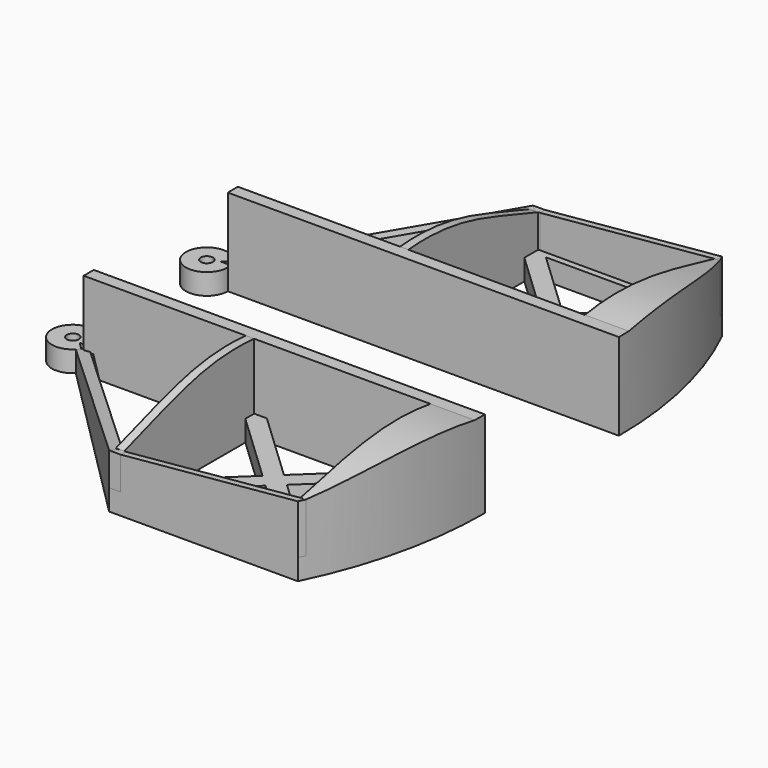
from build123d import *

# Parameters (mm, degrees)
F1_DEPTH       = 6.35
F2_R           = 1.8415
F3_DEPTH       = 25.4
F4_W           = 2.9205800795
F4_H           = 3.84
F5_DEPTH       = 20
F7_DEPTH       = 3.175
F9_DEPTH       = 1.905
F7_FACE_W      = 3.175
F7_FACE_H      = 10
F9_FACE_W      = 1.905
F9_FACE_H      = 10
F12_DEPTH      = 2.54
F16_END_RADIUS = 125
F15_W          = 3.84
F15_H          = 20
F16_REACH      = 136.0957238483
F18_DEPTH      = 15
F21_END_RADIUS = 125
F21_REACH      = 66.9646272281
F23_END_RADIUS = 125
F22_W          = 3.84
F22_H          = 20
F23_REACH      = 136.0957238483


with BuildPart() as f1:
    # F0 (on Top) → F1 (new body)
    with BuildSketch(Plane.XY):
        with BuildLine():
            Line((6.35, 0), (0, 0))
            Line((0, 0), (4.4901280605, 4.4901280605))
            ThreePointArc((4.4901280605, 4.4901280605), (-5.8666350314, -2.4300397955), (6.35, 0))
        make_face()
        with BuildLine():
            Line((4.4901280605, 4.4901280605), (0, 0))
            Line((0, 0), (6.35, 0))
            ThreePointArc((6.35, 0), (6.3162867067, 0.6534693866), (6.2155048065, 1.3))
            Line((6.2155048065, 1.3), (3.1384776311, 1.3))
            Line((3.1384776311, 1.3), (5.3142644127, 3.4757867817))
            ThreePointArc((5.3142644127, 3.4757867817), (4.9283617968, 4.0042165276), (4.4901280605, 4.4901280605))
        make_face()
        with BuildLine():
            Line((55, 55), (4.4901280605, 4.4901280605))
            ThreePointArc((4.4901280605, 4.4901280605), (4.9283617968, 4.0042165276), (5.3142644127, 3.4757867817))
            Line((5.3142644127, 3.4757867817), (55.5384776311, 53.7))
            Line((55.5384776311, 53.7), (110.9497216032, 53.7))
            Line((110.9497216032, 53.7), (110.9497216032, 1.3))
            Line((110.9497216032, 1.3), (55.5384776311, 1.3))
            Line((55.5384776311, 1.3), (6.2155048065, 1.3))
            ThreePointArc((6.2155048065, 1.3), (6.3162867067, 0.6534693866), (6.35, 0))
            Line((6.35, 0), (112.2497216032, 0))
            Line((112.2497216032, 0), (112.2497216032, 55))
            Line((112.2497216032, 55), (55, 55))
        make_face()
        with BuildLine():
            Line((55.5384776311, 53.7), (5.3142644127, 3.4757867817))
            ThreePointArc((5.3142644127, 3.4757867817), (5.8666350314, 2.4300397955), (6.2155048065, 1.3))
            Line((6.2155048065, 1.3), (55.5384776311, 1.3))
            Line((55.5384776311, 1.3), (55.5384776311, 53.7))
        make_face()
        Polygon((52.9984776311, 3.84), (9.2705800795, 3.84), (52.9984776311, 47.5678975516), align=None, mode=Mode.SUBTRACT)
        Polygon((83.2440996172, 27.5), (55.5384776311, 53.7), (55.5384776311, 1.3), align=None)
        Polygon((58.0784776311, 7.197828817), (58.0784776311, 47.802171183), (79.5473432911, 27.5), align=None, mode=Mode.SUBTRACT)
        Polygon((83.2440996172, 27.5), (55.5384776311, 1.3), (110.9497216032, 1.3), align=None)
        Polygon((104.5670003976, 3.84), (61.9211988367, 3.84), (83.2440996172, 24.0041385538), align=None, mode=Mode.SUBTRACT)
        Polygon((110.9497216032, 53.7), (55.5384776311, 53.7), (83.2440996172, 27.5), align=None)
        Polygon((83.2440996172, 30.9958614462), (61.9211988367, 51.16), (104.5670003976, 51.16), align=None, mode=Mode.SUBTRACT)
        Polygon((110.9497216032, 1.3), (110.9497216032, 53.7), (83.2440996172, 27.5), align=None)
        Polygon((108.4097216032, 7.197828817), (86.9408559432, 27.5), (108.4097216032, 47.802171183), align=None, mode=Mode.SUBTRACT)
        with BuildLine():
            Line((112.2497216032, 55), (112.2497216032, 0))
            Line((112.2497216032, 0), (125, 0))
            ThreePointArc((125, 0), (121.7707173347, 28.2292826653), (112.2497216032, 55))
        make_face()
    extrude(amount=F1_DEPTH)

    # F2 (on face) → F3 (cut)
    with BuildSketch(Plane.XY.offset(6.35)):
        Circle(F2_R)
    extrude(amount=-F3_DEPTH, mode=Mode.SUBTRACT)

    # F4 (on face) → F5 (join)
    with BuildSketch(Plane.XY.offset(6.35)):
        with Locations((7.8102900398, 1.92)):
            Rectangle(F4_W, F4_H)
    extrude(amount=F5_DEPTH)

    # F6 (on face) → F7 (join)
    with BuildSketch(Plane(origin=(0, 0, 0), x_dir=(-0.7071067812, -0.7071067812, 0), z_dir=(-0.7071067812, 0.7071067812, 0))):
        Polygon((-77.7817459305, 16.35), (-77.7817459305, 6.35), (-6.35, 6.35), align=None)
    extrude(amount=-F7_DEPTH)

    # F8 (on face) → F9 (join)
    with BuildSketch(Plane(origin=(0, 55, 0), x_dir=(-1, 0, 0), z_dir=(0, 1, 0))):
        Polygon((-112.2497216032, 21.35), (-112.2497216032, 6.35), (-58.5150640303, 6.35), (-58.5150640303, 16.35), align=None)
    extrude(amount=-F9_DEPTH)

    # F7_face (on face) → F10 section 0
    with BuildSketch(Plane(origin=(56.1225320151, 53.8774679849, 11.35), x_dir=(-0.7071067812, 0.7071067812, 0), z_dir=(0.7071067812, 0.7071067812, 0))):
        Rectangle(F7_FACE_W, F7_FACE_H)
    # F9_face (on face) → F10 section 1
    with BuildSketch(Plane(origin=(58.5150640303, 54.0475, 11.35), x_dir=(0, -1, 0), z_dir=(-1, 0, 0))):
        Rectangle(F9_FACE_W, F9_FACE_H)
    loft()

    # F11 (on face) → F12 (join)
    with BuildSketch(Plane.YZ.offset(58.0784776311)):
        with BuildLine():
            add(Edge.make_bspline(
                [(53.095, 16.35), (35.4615934193, 22.0014229417), (23.1343321502, 28.0265454203), (3.84, 26.35)],
                knots=[0, 0, 0, 0, 50.2598749004, 50.2598749004, 50.2598749004, 50.2598749004], degree=3))
            Line((3.84, 26.35), (3.84, 6.35))
            Line((3.84, 6.35), (7.197828817, 6.35))
            Line((7.197828817, 6.35), (47.802171183, 6.35))
            Line((47.802171183, 6.35), (53.095, 6.35))
            Line((53.095, 6.35), (53.095, 16.35))
        make_face()
    extrude(amount=-F12_DEPTH)


with BuildPart() as f14_1:
    # F14: instance of F1
    add(f1.part.mirror(Plane(origin=(61.5116499252, -25.4, 4.122937651), x_dir=(1, 0, 0), z_dir=(0, -1, 0))))

    # F17 (on face) → F18 (join, through all)
    with BuildSketch(Plane.XY.offset(6.35)):
        with BuildLine():
            Line((113.1632492243, -103.895), (112.2497216032, -103.895))
            Line((112.2497216032, -103.895), (112.2497216032, -105.8))
            ThreePointArc((112.2497216032, -105.8), (112.7105102046, -104.8494300565), (113.1632492243, -103.895))
        make_face()
    extrude(amount=F18_DEPTH)

    f21_end = (Plane(origin=(0, -50.8, 10.675), x_dir=(-1, 0, 0), z_dir=(0, 0, -1)) * Cylinder(F21_END_RADIUS, 552.5885115546, mode=Mode.PRIVATE)).faces().sort_by_distance((122.0049305418, -77.9992081407, 5.7463948228))[0]
    # F20 (on offset) → F21 (join, up to the whole of a round face its end follows)
    with BuildSketch(Plane(origin=(111.5847216032, 0, 0), x_dir=(0, -1, 0), z_dir=(-1, 0, 0))):
        with BuildLine():
            Line((103.895, 6.35), (103.895, 21.35))
            add(Edge.make_bspline(
                [(103.895, 21.35), (87.9248529673, 25.0397752971), (72.7827176452, 29.3548926711), (54.64, 26.35)],
                knots=[0, 0, 0, 0, 49.5081308979, 49.5081308979, 49.5081308979, 49.5081308979], degree=3))
            Line((54.64, 26.35), (54.64, 6.35))
            Line((54.64, 6.35), (103.895, 6.35))
        make_face()
    f21_long = extrude(amount=-F21_REACH, mode=Mode.PRIVATE)
    add(split(f21_long, bisect_by=f21_end, keep=Keep.BOTTOM, mode=Mode.PRIVATE))

    f23_end = (Plane(origin=(0, -50.8, 13.7255002307), x_dir=(-1, 0, 0), z_dir=(0, 0, -1)) * Cylinder(F23_END_RADIUS, 691.0373274131, mode=Mode.PRIVATE)).faces().sort_by_distance((121.7707173347, -79.0292826653, 13.7255002307))[0]
    # F22 (on face) → F23 (join, up to the whole of a round face its end follows)
    with BuildSketch(Plane.YZ.offset(9.2705800795)):
        with Locations((-52.72, 16.35)):
            Rectangle(F22_W, F22_H)
    f23_long = extrude(amount=F23_REACH, mode=Mode.PRIVATE)
    add(split(f23_long, bisect_by=f23_end, keep=Keep.BOTTOM, mode=Mode.PRIVATE))


with BuildPart() as f1_1:
    add(f1.part)

    f16_end = (Plane(origin=(0, 0, 3.175), x_dir=(-1, 0, 0), z_dir=(0, 0, -1)) * Cylinder(F16_END_RADIUS, 690.8507047952, mode=Mode.PRIVATE)).faces().sort_by_distance((121.7707173347, 28.2292826653, 3.175))[0]
    # F15 (on face) → F16 (join, up to the whole of a round face its end follows)
    with BuildSketch(Plane.YZ.offset(9.2705800795)):
        with Locations((1.92, 16.35)):
            Rectangle(F15_W, F15_H)
    f16_long = extrude(amount=F16_REACH, mode=Mode.PRIVATE)
    add(split(f16_long, bisect_by=f16_end, keep=Keep.BOTTOM, mode=Mode.PRIVATE))

    # F24: F14_1 across plane
    add(f14_1.part.mirror(Plane(origin=(61.5116499252, -25.4, 4.122937651), x_dir=(1, 0, 0), z_dir=(0, -1, 0))))


solid = Compound([f14_1.part, f1_1.part])
